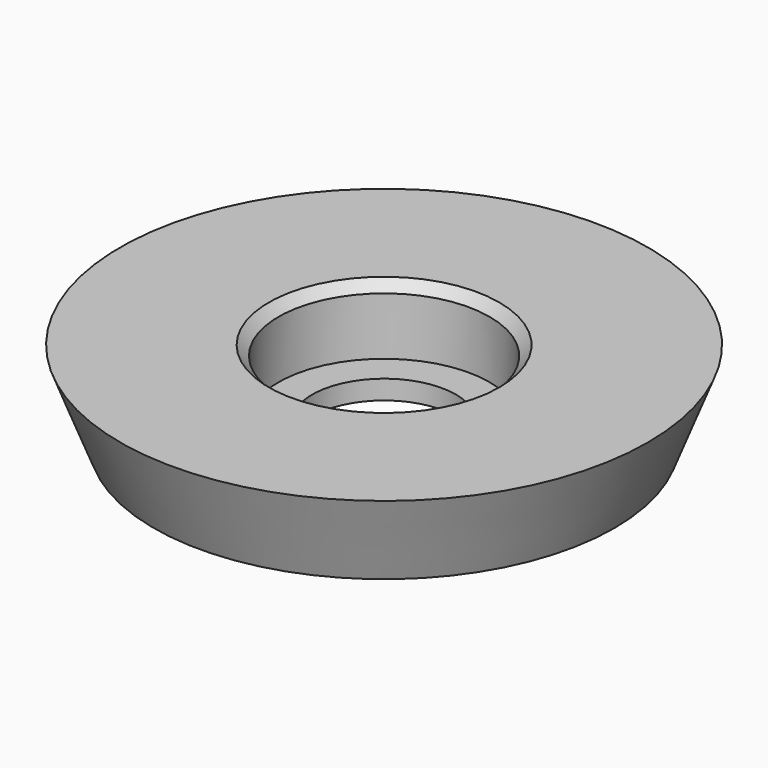
from build123d import *

# Parameters (mm, degrees)
F0_R     = 27.5
F0_R_2   = 7.5
F1_DEPTH = 2
F2_R     = 27.5
F2_R_2   = 11
F3_DEPTH = 7
F4_SIZE2 = 3.49999
F4_SIZE  = 8.99999
F5_SIZE  = 1


# Not quite as in the source:
# - a fillet or chamfer is up to 0.001 mm smaller than in the source, because OpenCascade refuses the exact size


with BuildPart() as f1:
    # F0 (on Top) → F1 (new body)
    with BuildSketch(Plane.XY):
        Circle(F0_R)
        Circle(F0_R_2, mode=Mode.SUBTRACT)
    extrude(amount=F1_DEPTH)

    # F2 (on face) → F3 (join)
    with BuildSketch(Plane.XY.offset(2)):
        Circle(F2_R)
        Circle(F2_R_2, mode=Mode.SUBTRACT)
    extrude(amount=F3_DEPTH)

    # F4 (size 9 and 3.5 in the source; OpenCascade refuses exactly that, so slightly less here)
    f4_edges = [f1.edges().sort_by_distance(p)[0] for p in [
        (-27.5, 0, 0),
    ]]
    f4_side = f1.faces().sort_by_distance((-27.5, 0, 4.5))[0]
    chamfer(f4_edges, length=F4_SIZE, length2=F4_SIZE2, reference=f4_side)

    # F5
    f5_edges = [f1.edges().sort_by_distance(p)[0] for p in [
        (-11, 0, 9),
    ]]
    chamfer(f5_edges, length=F5_SIZE)


solid = f1.part
